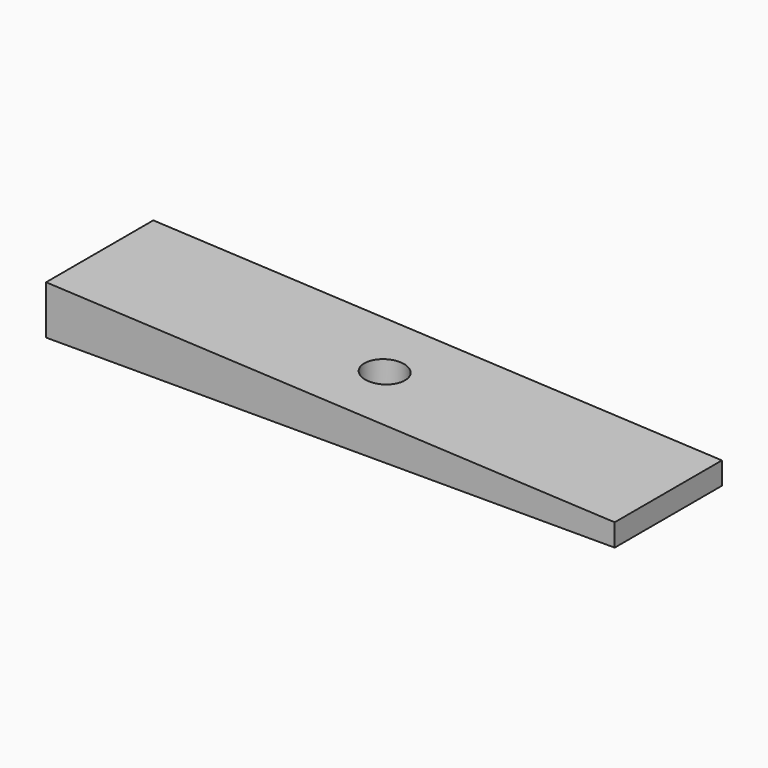
from build123d import *

# Parameters (mm, degrees)
F0_W        = 140
F0_H        = 33
F0_R        = 5
F1_DEPTH    = 12
F2_T1_DEPTH = 760.9710283957


# Not quite as in the source:
# - a fillet or chamfer that OpenCascade refuses, or shapes differently, is made with other operations: its cross-section is extruded or revolved along the edge and cut away or added


with BuildPart() as f1:
    # F0 (on Top) → F1 (new body)
    with BuildSketch(Plane.XY):
        with Locations((-0.2143342793, 0.0709771141)):
            Rectangle(F0_W, F0_H)
        Circle(F0_R, mode=Mode.SUBTRACT)
    extrude(amount=F1_DEPTH)

    # F2: chamfer of 6.5 x 140 on 1 edges, made by hand

    # F2_s2 → F2_t1 (cut)
    with BuildSketch(Plane.XZ.offset(-380.556491312)):
        Polygon((69.7856657207, 5.5), (-70.2143342793, 12), (69.7856657207, 12), align=None)
    extrude(amount=F2_T1_DEPTH, mode=Mode.SUBTRACT)


solid = f1.part
